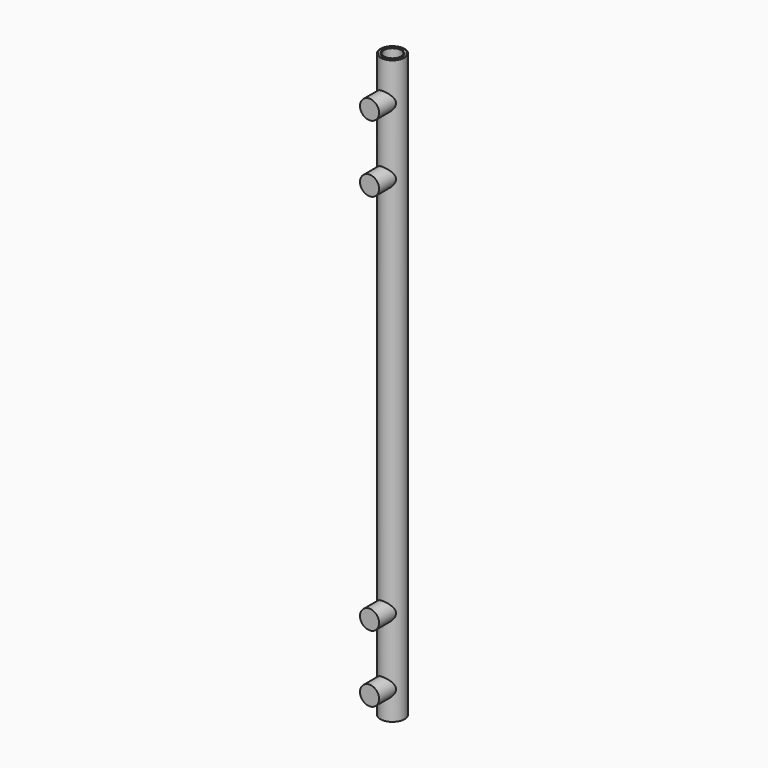
from build123d import *

# Parameters (mm, degrees)
F0_R     = 6.35
F1_DEPTH = 304.8
F2_R     = 5
F4_DEPTH = 15
F3_R     = 4.445
F5_DEPTH = 304.8010001


# Not quite as in the source:
# - a pattern or mirror of a feature is missing from the dataset's text; its kind, count and spacing are read off the source's solid


with BuildPart() as f1:
    # F0 (on Top) → F1 (new body)
    with BuildSketch(Plane.XY):
        Circle(F0_R)
    extrude(amount=F1_DEPTH)

    # F2 (on Front) → F4 (join)
    with BuildSketch(Plane.XZ):
        with Locations((0, 15)):
            Circle(F2_R)
        with Locations((0, 50)):
            Circle(F2_R)
        with Locations((0, 250)):
            Circle(F2_R)
        with Locations((0, 285)):
            Circle(F2_R)
    extrude(amount=F4_DEPTH)

    # F3 (on face) → F5 (cut, through all)
    with BuildSketch(Plane.XY.offset(304.8)):
        Circle(F3_R)
    extrude(amount=-F5_DEPTH, mode=Mode.SUBTRACT)

    # F8: sweep along a path in F6
    with BuildLine(Plane.XY.offset(304.8)) as f8_path:
        CenterArc((0, 0), 5.461, 0, 360)
    # F7 (on Front) → F8 (sweep, cut)
    with BuildSketch(Plane.XZ):
        with BuildLine():
            Line((-5, 304.8), (-6, 304.8))
            ThreePointArc((-6, 304.8), (-5.5, 304.3), (-5, 304.8))
        make_face()
    f8 = sweep(path=f8_path.line, mode=Mode.SUBTRACT)

    # F8_copies: F8 across plane
    add(f8.mirror(Plane(origin=(0, 0, 152.4), x_dir=(-1, 0, 0), z_dir=(0, 0, -1))), mode=Mode.SUBTRACT)


solid = f1.part
